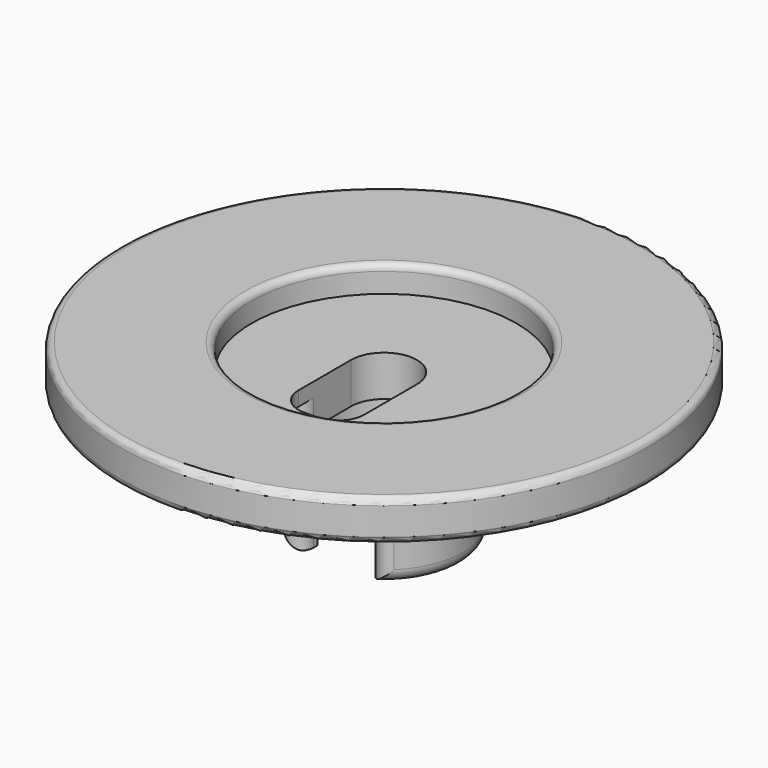
from build123d import *

# Parameters (mm, degrees)
F0_R           = 20.05
F1_DEPTH       = 3.1
F2_R           = 10.05
F3_DEPTH       = 2
F4_R           = 0.5
F6_R           = 6
F7_DEPTH       = 10
F8_R           = 4.05
F9_DEPTH       = 8
F10_DEPTH      = 10.001
F10_DEPTH_BACK = 3.1010001
F11_T1_DEPTH   = 15.3170452501
F11_T4_ANGLE   = 359.9586190749


# Not quite as in the source:
# - a fillet or chamfer that OpenCascade refuses, or shapes differently, is made with other operations: its cross-section is extruded or revolved along the edge and cut away or added


with BuildPart() as f1:
    # F0 (on Top) → F1 (new body)
    with BuildSketch(Plane.XY):
        Circle(F0_R)
    extrude(amount=F1_DEPTH)

    # F2 (on face) → F3 (cut)
    with BuildSketch(Plane.XY.offset(3.1)):
        Circle(F2_R)
    extrude(amount=-F3_DEPTH, mode=Mode.SUBTRACT)

    # F4
    f4_edges = [f1.edges().sort_by_distance(p)[0] for p in [
        (-20.05, 0, 3.1),
        (-10.05, 0, 3.1),
        (-20.05, 0, 0),
    ]]
    fillet(f4_edges, radius=F4_R)

    # F6 (on face) → F7 (join)
    with BuildSketch(Plane(origin=(0, 0, 0), x_dir=(1, 0, 0), z_dir=(0, 0, -1))):
        Circle(F6_R)
    extrude(amount=F7_DEPTH)

    # F8 (on face) → F9 (cut)
    with BuildSketch(Plane(origin=(0, 0, -10), x_dir=(1, 0, 0), z_dir=(0, 0, -1))):
        Circle(F8_R)
    extrude(amount=-F9_DEPTH, mode=Mode.SUBTRACT)

    # F5 (on face) → F10 (cut, two sides)
    with BuildSketch(Plane(origin=(0, 0, 0), x_dir=(1, 0, 0), z_dir=(0, 0, -1))) as f10_sk:
        with BuildLine():
            Line((-2.5, 5), (-2.5, 0))
            ThreePointArc((-2.5, 0), (0, -2.5), (2.5, 0))
            Line((2.5, 0), (2.5, 5))
            ThreePointArc((2.5, 5), (1.9142135624, 6.4142135624), (0.5, 7))
            Line((0.5, 7), (-0.5, 7))
            ThreePointArc((-0.5, 7), (-1.9142135624, 6.4142135624), (-2.5, 5))
        make_face()
    extrude(amount=F10_DEPTH, mode=Mode.SUBTRACT)
    extrude(f10_sk.sketch, amount=-F10_DEPTH_BACK, mode=Mode.SUBTRACT)

    # F11: fillet of radius 1 on 3 edges, made by hand

    # F11_s2 → F11_t1 (cut)
    with BuildSketch(Plane.XY.offset(-15.3170452501)):
        with BuildLine():
            ThreePointArc((-4.2, -4.2848570571), (-3.1127016654, -4.49266866), (-2.5, -3.5707142143))
            Line((-2.5, -3.5707142143), (-2.4, -3.5707142143))
            ThreePointArc((-2.4, -3.5707142143), (-2.4, -5), (-2.3442646941, -5.4568235306))
            Line((-2.3442646941, -5.4568235306), (-2.4820201112, -5.5722146555))
            ThreePointArc((-2.4820201112, -5.5722146555), (-3.4303168121, -5.0440981918), (-4.27, -4.3562713414))
            Line((-4.27, -4.3562713414), (-4.2, -4.2848570571))
        make_face()
        with BuildLine():
            ThreePointArc((4.2, -4.2848570571), (3.1127016654, -4.49266866), (2.5, -3.5707142143))
            Line((2.5, -3.5707142143), (2.4, -3.5707142143))
            ThreePointArc((2.4, -3.5707142143), (2.4, -5), (2.3442646941, -5.4568235306))
            Line((2.3442646941, -5.4568235306), (2.4820201112, -5.5722146555))
            ThreePointArc((2.4820201112, -5.5722146555), (3.4303168121, -5.0440981918), (4.27, -4.3562713414))
            Line((4.27, -4.3562713414), (4.2, -4.2848570571))
        make_face()
    extrude(amount=F11_T1_DEPTH, mode=Mode.SUBTRACT)

    # F11_s3 → F11_t4 (revolve, cut)
    with BuildSketch(Plane(origin=(0, 0, 0), x_dir=(0, 0, 1), z_dir=(-0.9999999348, -0.0003611167, 0))):
        with BuildLine():
            ThreePointArc((-10, -5), (-9.7071067812, -5.7071067812), (-9, -6))
            Line((-9, -6), (-10, -6))
            Line((-10, -6), (-10, -5))
        make_face()
    revolve(axis=Axis((0, 0, -10), (0, 0, 1)), revolution_arc=F11_T4_ANGLE, mode=Mode.SUBTRACT)


solid = f1.part
